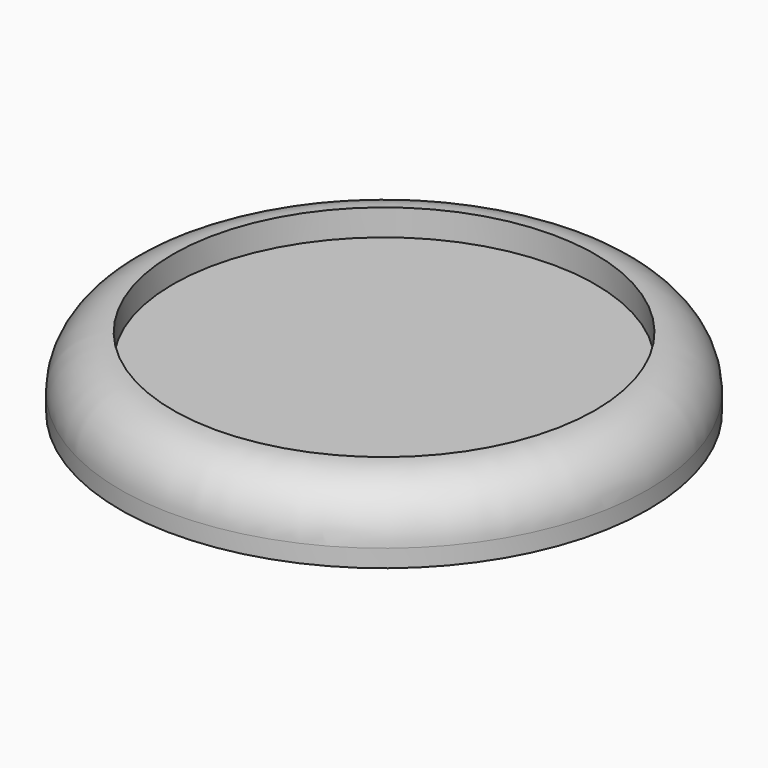
from build123d import *

# Parameters (mm, degrees)
F0_R     = 15
F1_DEPTH = 4
F2_R     = 3
F3_DEPTH = 1.5
F4_T     = -1
F5_DEPTH = 1.5


with BuildPart() as f1:
    # F0 (on Top) → F1 (new body)
    with BuildSketch(Plane.XY):
        Circle(F0_R)
    extrude(amount=F1_DEPTH)

    # F2
    f2_edges = [f1.edges().sort_by_distance(p)[0] for p in [
        (-15, 0, 4),
    ]]
    fillet(f2_edges, radius=F2_R)

    # F3 (cut): a face of the model
    f3_faces = [f1.faces().sort_by_distance(p)[0] for p in [
        (0, 0, 4),
    ]]
    extrude(f3_faces, amount=-F3_DEPTH, mode=Mode.SUBTRACT)

    # F4
    f4_openings = [f1.faces().sort_by_distance(p)[0] for p in [
        (0, 0, 0),
    ]]
    offset(amount=F4_T, openings=f4_openings, kind=Kind.INTERSECTION)

    # F5 (add): a face of the model
    f5_faces = [f1.faces().sort_by_distance(p)[0] for p in [
        (0, 0, 1.5),
    ]]
    extrude(f5_faces, amount=F5_DEPTH)


solid = f1.part
